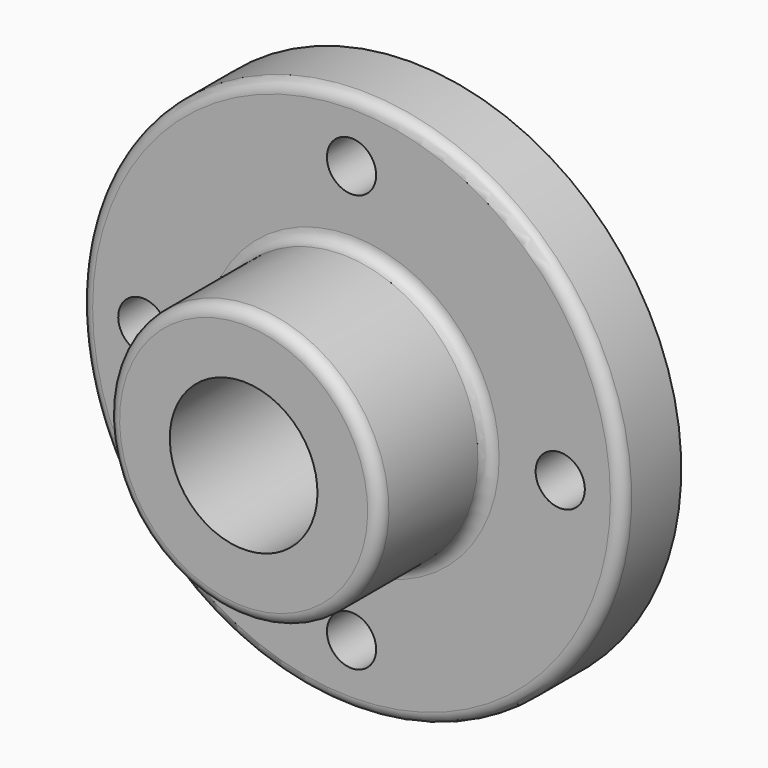
from build123d import *

# Parameters (mm, degrees)
F2_R            = 3.048
F3_R            = 6.35
F4_DEPTH        = 19.051
F4_COPIES_COUNT = 4


# Not quite as in the source:
# - a pattern or mirror of a feature is missing from the dataset's text; its kind, count and spacing are read off the source's solid


with BuildPart() as f1:
    # F0 (on Right) → F1 (revolve)
    with BuildSketch(Plane.YZ):
        Polygon((0, 19.05), (53.848, 19.05), (53.848, 69.85), (34.798, 69.85), (34.798, 35.052), (0, 35.052), align=None)
    revolve(axis=Axis((0, 33.935634885, 0), (0, 1, 0)))

    # F2
    f2_edges = [f1.edges().sort_by_distance(p)[0] for p in [
        (0, 34.798, -69.85),
        (0, 34.798, -35.052),
        (0, 0, -35.052),
    ]]
    fillet(f2_edges, radius=F2_R)

    # F3 (on face) → F4 (cut, through all)
    with BuildSketch(Plane.XZ.offset(-34.798)):
        with Locations((0, 53.848)):
            Circle(F3_R)
    f4 = extrude(amount=-F4_DEPTH, mode=Mode.SUBTRACT)

    # F4_copies: F4 ×4 about axis
    f4_copies_axis = Axis((0, 0, 0), (0, 1, 0))
    for i in range(1, F4_COPIES_COUNT):
        add(f4.rotate(f4_copies_axis, i * 360 / F4_COPIES_COUNT), mode=Mode.SUBTRACT)


solid = f1.part
